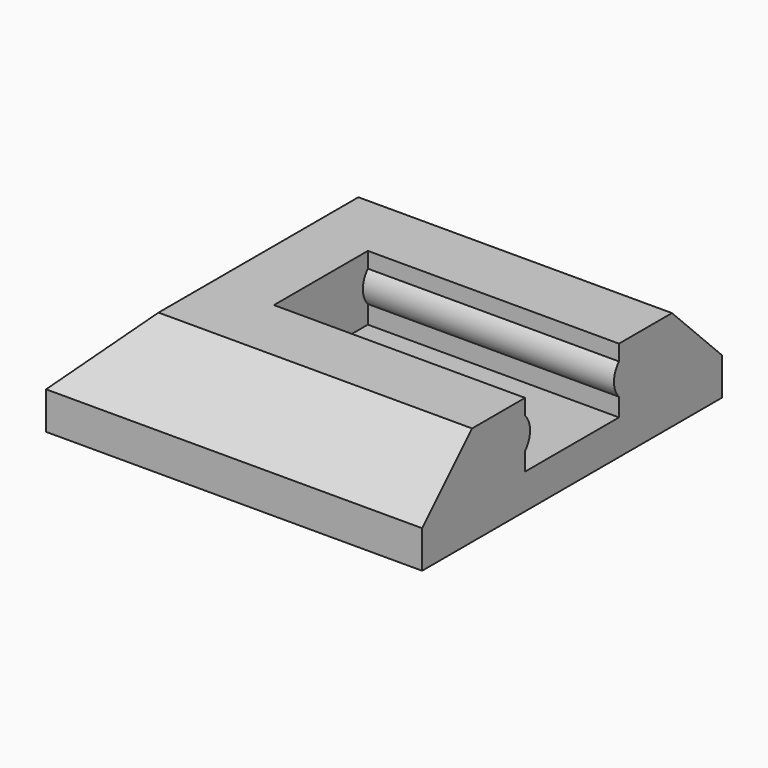
from build123d import *

# Parameters (mm, degrees)
F0_W      = 16
F0_H      = 6
F1_DEPTH  = 95
F2_DEPTH  = 5
F3_R      = 2
F4_DEPTH  = 127.001
F5_SIZE   = 0.49999
F6_DEPTH  = 25
F8_DEPTH  = 25
F9_W      = 318.6057507992
F9_H      = 243.2989366353
F10_DEPTH = 19.501
F12_DEPTH = 10
F14_DEPTH = 8.001
F15_SIZE  = 5
F16_SIZE  = 5


# Not quite as in the source:
# - a fillet or chamfer is up to 0.001 mm smaller than in the source, because OpenCascade refuses the exact size


with BuildPart() as f1:
    # F0 (on Top) → F1 (new body)
    with BuildSketch(Plane.XY):
        Polygon((-8, -4.5), (63.5, -4.5), (63.5, 4.5), (-26, 4.5), (-28, 4.5), (-44, 4.5), (-46, 4.5), (-63.5, 4.5), (-63.5, -4.5), (-28, -4.5), (-26, -4.5), (-10, -4.5), align=None)
        with Locations((-54, 0)):
            Rectangle(F0_W, F0_H, mode=Mode.SUBTRACT)
        with Locations((-36, 0)):
            Rectangle(F0_W, F0_H, mode=Mode.SUBTRACT)
        with Locations((-18, 0)):
            Rectangle(F0_W, F0_H, mode=Mode.SUBTRACT)
        Rectangle(F0_W, F0_H, mode=Mode.SUBTRACT)
        with Locations((18, 0)):
            Rectangle(F0_W, F0_H, mode=Mode.SUBTRACT)
        with Locations((36, 0)):
            Rectangle(F0_W, F0_H, mode=Mode.SUBTRACT)
        with Locations((54, 0)):
            Rectangle(F0_W, F0_H, mode=Mode.SUBTRACT)
    extrude(amount=F1_DEPTH)

    # F0 (on Top) → F2 (join)
    with BuildSketch(Plane.XY):
        Polygon((-8, -4.5), (63.5, -4.5), (63.5, 4.5), (-26, 4.5), (-28, 4.5), (-44, 4.5), (-46, 4.5), (-63.5, 4.5), (-63.5, -4.5), (-28, -4.5), (-26, -4.5), (-10, -4.5), align=None)
        with Locations((-54, 0)):
            Rectangle(F0_W, F0_H, mode=Mode.SUBTRACT)
        with Locations((-36, 0)):
            Rectangle(F0_W, F0_H, mode=Mode.SUBTRACT)
        with Locations((-18, 0)):
            Rectangle(F0_W, F0_H, mode=Mode.SUBTRACT)
        Rectangle(F0_W, F0_H, mode=Mode.SUBTRACT)
        with Locations((18, 0)):
            Rectangle(F0_W, F0_H, mode=Mode.SUBTRACT)
        with Locations((36, 0)):
            Rectangle(F0_W, F0_H, mode=Mode.SUBTRACT)
        with Locations((54, 0)):
            Rectangle(F0_W, F0_H, mode=Mode.SUBTRACT)
        with Locations((-54, 0)):
            Rectangle(F0_W, F0_H)
        with Locations((-36, 0)):
            Rectangle(F0_W, F0_H)
        with Locations((-18, 0)):
            Rectangle(F0_W, F0_H)
        Rectangle(F0_W, F0_H)
        with Locations((18, 0)):
            Rectangle(F0_W, F0_H)
        with Locations((36, 0)):
            Rectangle(F0_W, F0_H)
        with Locations((54, 0)):
            Rectangle(F0_W, F0_H)
    extrude(amount=-F2_DEPTH)

    # F3 (on face) → F4 (cut, through all)
    with BuildSketch(Plane(origin=(-63.5, 0, 0), x_dir=(0, -1, 0), z_dir=(-1, 0, 0))):
        with Locations((-6, -2.5)):
            Circle(F3_R)
        with Locations((6, -2.5)):
            Circle(F3_R)
    extrude(amount=-F4_DEPTH, mode=Mode.SUBTRACT)

    # F5 (size 0.5 in the source; OpenCascade refuses exactly that, so slightly less here)
    f5_edges = [f1.edges().sort_by_distance(p)[0] for p in [
        (-63.5, 4.5, 46.911438),
        (-63.5, -4.5, 46.911438),
        (0, 4.5, -5),
        (-63.5, 0, -5),
        (-63.5, 4, -2.5),
        (0, 4.5, 95),
        (-63.5, 0, 95),
        (0, -4.5, 95),
        (63.5, 0, 95),
        (63.5, 0, -5),
        (63.5, 4.5, 46.911438),
        (63.5, -4.5, 46.911438),
        (-63.5, -4, -2.5),
        (63.5, 4, -2.5),
        (63.5, -4, -2.5),
        (54, -3, 95),
        (46, 0, 95),
        (54, 3, 95),
        (62, 0, 95),
        (44, 0, 95),
        (36, 3, 95),
        (36, -3, 95),
        (8, 0, 95),
        (10, 0, 95),
        (18, 3, 95),
        (18, -3, 95),
        (26, 0, 95),
        (28, 0, 95),
        (0, 3, 95),
        (0, -3, 95),
        (-8, 0, 95),
        (-10, 0, 95),
        (-18, -3, 95),
        (-26, 0, 95),
        (-18, 3, 95),
        (-36, 3, 95),
        (-28, 0, 95),
        (-36, -3, 95),
        (-54, 3, 95),
        (-62, 0, 95),
        (-54, -3, 95),
        (-46, 0, 95),
        (-44, 0, 95),
    ]]
    chamfer(f5_edges, length=F5_SIZE)

    # F3 (on face) → F6 (join)
    with BuildSketch(Plane(origin=(-63.5, 0, 0), x_dir=(0, -1, 0), z_dir=(-1, 0, 0))):
        with BuildLine():
            ThreePointArc((-4.5, -1.1771243445), (-4.1291713066, -1.7928932188), (-4, -2.5))
            ThreePointArc((-4, -2.5), (-4.1291713066, -3.2071067812), (-4.5, -3.8228756555))
            Line((-4.5, -3.8228756555), (-4.5, -5))
            Line((-4.5, -5), (4.5, -5))
            Line((4.5, -5), (4.5, -3.8228756555))
            ThreePointArc((4.5, -3.8228756555), (4, -2.5), (4.5, -1.1771243445))
            Line((4.5, -1.1771243445), (4.5, 95))
            Line((4.5, 95), (-4.5, 95))
            Line((-4.5, 95), (-4.5, -1.1771243445))
        make_face()
    extrude(amount=F6_DEPTH)


with BuildPart() as f8:
    # F7 (on face) → F8 (new body)
    with BuildSketch(Plane(origin=(-88.5, 0, 0), x_dir=(0, -1, 0), z_dir=(-1, 0, 0))):
        with BuildLine():
            Line((15, 0), (4.7, 0))
            Line((4.7, 0), (4.7, -1.2550100402))
            ThreePointArc((4.7, -1.2550100402), (4.2, -2.5), (4.7, -3.7449899598))
            Line((4.7, -3.7449899598), (4.7, -5.2))
            Line((4.7, -5.2), (-4.7, -5.2))
            Line((-4.7, -5.2), (-4.7, -3.7449899598))
            ThreePointArc((-4.7, -3.7449899598), (-4.2, -2.5), (-4.7, -1.2550100402))
            Line((-4.7, -1.2550100402), (-4.7, 0))
            Line((-4.7, 0), (-15, 0))
            Line((-15, 0), (-15, -8))
            Line((-15, -8), (15, -8))
            Line((15, -8), (15, 0))
        make_face()
    extrude(amount=F8_DEPTH)


with BuildPart() as f10_tool:
    # F9 (on face) → F10 (new body, through all)
    with BuildSketch(Plane(origin=(0, 4.5, 0), x_dir=(-1, 0, 0), z_dir=(0, 1, 0))):
        with Locations((-68.3380588889, 100.3342196345)):
            Rectangle(F9_W, F9_H)
    extrude(amount=-F10_DEPTH)


with BuildPart() as f1_1:
    add(f1.part)

    # F10: cut by f10_tool
    add(f10_tool.part, mode=Mode.SUBTRACT)


with BuildPart() as f8_1:
    add(f8.part)

    # F10: cut by f10_tool
    add(f10_tool.part, mode=Mode.SUBTRACT)

    # F11 (on face) → F12 (join)
    with BuildSketch(Plane(origin=(-113.5, 0, 0), x_dir=(0, -1, 0), z_dir=(-1, 0, 0))):
        with BuildLine():
            Line((-4.7, -1.2550100402), (-4.7, 0))
            Line((-4.7, 0), (-15, 0))
            Line((-15, 0), (-15, -8))
            Line((-15, -8), (15, -8))
            Line((15, -8), (15, 0))
            Line((15, 0), (4.7, 0))
            Line((4.7, 0), (4.7, -1.2550100402))
            ThreePointArc((4.7, -1.2550100402), (4.2, -2.5), (4.7, -3.7449899598))
            Line((4.7, -3.7449899598), (4.7, -5.2))
            Line((4.7, -5.2), (-4.7, -5.2))
            Line((-4.7, -5.2), (-4.7, -3.7449899598))
            ThreePointArc((-4.7, -3.7449899598), (-4.2, -2.5), (-4.7, -1.2550100402))
        make_face()
        with BuildLine():
            Line((4.7, 0), (-4.7, 0))
            Line((-4.7, 0), (-4.7, -1.2550100402))
            ThreePointArc((-4.7, -1.2550100402), (-4.2, -2.5), (-4.7, -3.7449899598))
            Line((-4.7, -3.7449899598), (-4.7, -5.2))
            Line((-4.7, -5.2), (4.7, -5.2))
            Line((4.7, -5.2), (4.7, -3.7449899598))
            ThreePointArc((4.7, -3.7449899598), (4.2, -2.5), (4.7, -1.2550100402))
            Line((4.7, -1.2550100402), (4.7, 0))
        make_face()
    extrude(amount=F12_DEPTH)

    # F13 (on face) → F14 (cut, through all)
    with BuildSketch(Plane(origin=(0, 0, -8), x_dir=(1, 0, 0), z_dir=(0, 0, -1))):
        Polygon((-93.395665288, -19.6107532829), (-75.3739327192, -19.6107532829), (-75.3739327192, 58.0060165375), (-93.395665288, 58.0060165375), (-93.395665288, 15), (-90.9648165107, 15), (-90.9648165107, -4.5), (-88.5, -4.5), (-88.5, -15), (-93.395665288, -15), align=None)
        Polygon((-93.395665288, 15), (-93.395665288, -15), (-88.5, -15), (-88.5, -4.5), (-90.9648165107, -4.5), (-90.9648165107, 15), align=None)
    extrude(amount=-F14_DEPTH, mode=Mode.SUBTRACT)

    # F15
    f15_edges = [f8_1.edges().sort_by_distance(p)[0] for p in [
        (-108.447833, 15, 0),
        (-108.447833, -15, 0),
    ]]
    chamfer(f15_edges, length=F15_SIZE)

    # F16
    f16_edges = [f8_1.edges().sort_by_distance(p)[0] for p in [
        (-123.5, 0, 0),
    ]]
    chamfer(f16_edges, length=F16_SIZE)


solid = f8_1.part
